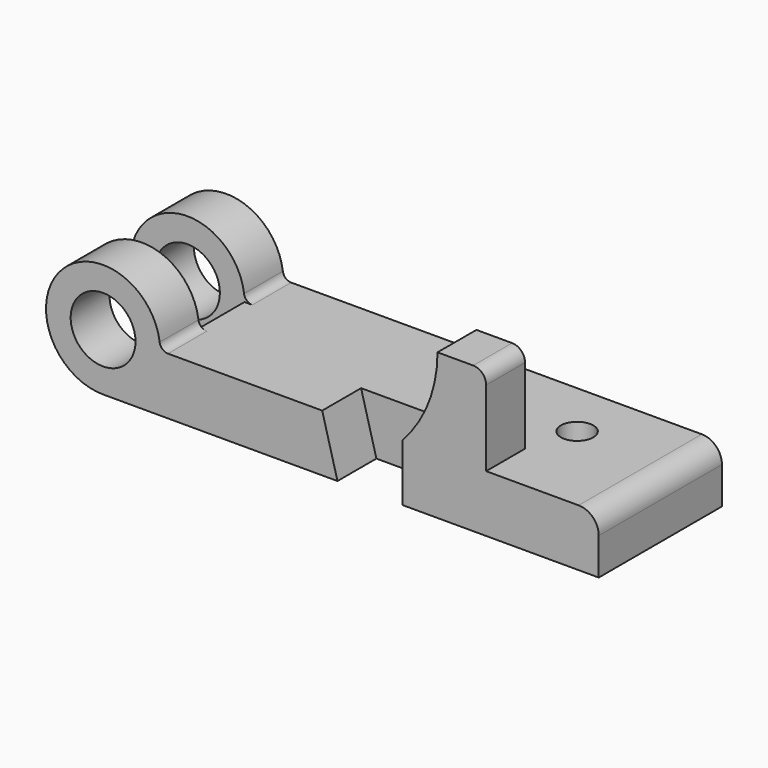
from build123d import *

# Parameters (mm, degrees)
F0_R     = 12.7
F1_DEPTH = 60.325
F3_W     = 32.8422
F3_H     = 41.275
F6_DEPTH = 34.798
F7_DEPTH = 19.05
F5_W     = 50.4518977821
F5_H     = 22.3266
F5_R     = 6.35
F8_DEPTH = 47.498
F9_R     = 3.302


with BuildPart() as f1:
    # F0 (on Front) → F1 (new body)
    with BuildSketch(Plane.XZ):
        with BuildLine():
            ThreePointArc((-79.7361564685, 22.352), (-117.8934072416, 38.1572507731), (-102.0881564685, 0))
            Line((-102.0881564685, 0), (92.1202435315, 0))
            Line((92.1202435315, 0), (92.1202435315, 14.478))
            ThreePointArc((92.1202435315, 14.478), (89.8140023266, 20.0457587951), (84.2462435315, 22.352))
            Line((84.2462435315, 22.352), (48.0004435315, 22.352))
            Line((48.0004435315, 22.352), (48.0004435315, 52.07))
            ThreePointArc((48.0004435315, 52.07), (46.5125459799, 55.6621024484), (42.9204435315, 57.15))
            Line((42.9204435315, 57.15), (28.9504435315, 57.15))
            ThreePointArc((28.9504435315, 57.15), (25.3762588931, 38.4343576341), (15.1582435315, 22.352))
            Line((15.1582435315, 22.352), (-79.7361564685, 22.352))
        make_face()
        with Locations((-102.0881564685, 22.352)):
            Circle(F0_R, mode=Mode.SUBTRACT)
    extrude(amount=-F1_DEPTH)

    # F3 (on offset) → F6 (cut, through all)
    with BuildSketch(Plane.XY.offset(22.352)):
        with Locations((31.5793435315, 39.6875)):
            Rectangle(F3_W, F3_H)
    extrude(amount=F6_DEPTH, mode=Mode.SUBTRACT)

    # F4 (on Front) → F7 (cut)
    with BuildSketch(Plane.XZ):
        Polygon((15.1582435315, 0), (15.1582435315, 22.352), (-16.2361564685, 22.352), (-10.2417564685, 0), align=None)
    extrude(amount=-F7_DEPTH, mode=Mode.SUBTRACT)

    # F5 (on offset) → F8 (cut, symmetric)
    with BuildSketch(Plane.XY.offset(22.352)):
        with Locations((-104.9621053595, 30.1625)):
            Rectangle(F5_W, F5_H)
        with Locations((53.2582435315, 37.973)):
            Circle(F5_R)
    extrude(amount=F8_DEPTH, both=True, mode=Mode.SUBTRACT)

    # F9
    f9_edges = [f1.edges().sort_by_distance(p)[0] for p in [
        (-79.736156, 9.4996, 22.352),
        (-79.736156, 50.8254, 22.352),
    ]]
    fillet(f9_edges, radius=F9_R)


solid = f1.part
